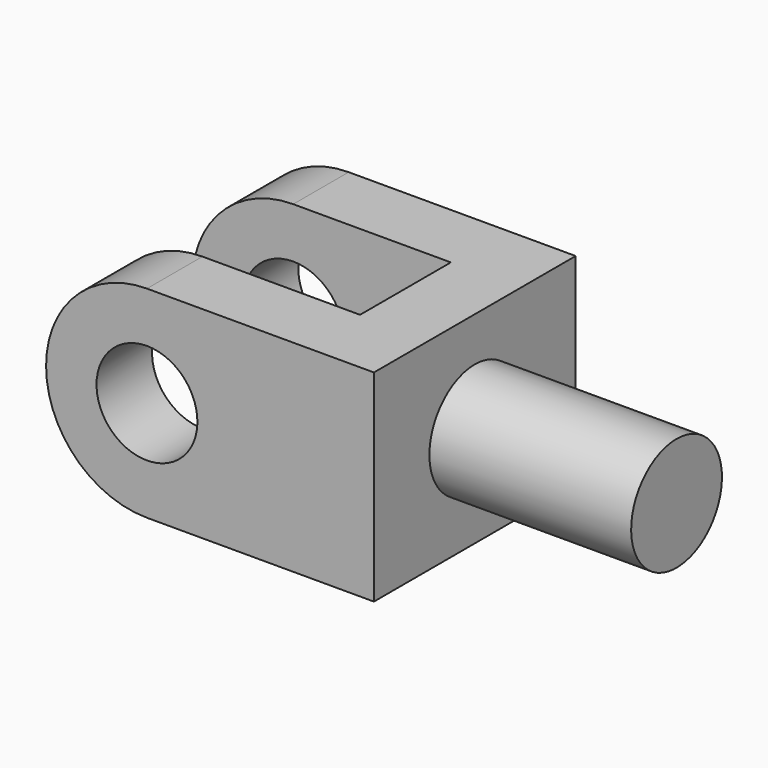
from build123d import *

# Parameters (mm, degrees)
F1_DEPTH = 812.8
F3_DEPTH = 1016.001
F4_R     = 406.4
F5_R     = 406.39999
F7_DEPTH = 812.8


# Not quite as in the source:
# - a fillet or chamfer is up to 0.001 mm smaller than in the source, because OpenCascade refuses the exact size


with BuildPart() as f1:
    # F0 (on Top) → F1 (new body)
    with BuildSketch(Plane.XY):
        Polygon((1205.200382638, 51.7077632248), (-115.599617362, 51.7077632248), (-115.599617362, -227.6922367752), (925.800382638, -227.6922367752), (925.800382638, -684.8922367752), (-115.599617362, -684.8922367752), (-115.599617362, -964.2922367752), (1205.200382638, -964.2922367752), (1205.200382638, -227.6922367752), align=None)
    extrude(amount=-F1_DEPTH)

    # F2 (on face) → F3 (cut, through all)
    with BuildSketch(Plane.XZ.offset(964.2922367752)):
        with BuildLine():
            ThreePointArc((494.000382638, -406.4), (434.4844805751, -262.7159020629), (290.800382638, -203.2))
            ThreePointArc((290.800382638, -203.2), (147.1162847009, -550.0840979371), (494.000382638, -406.4))
        make_face()
    extrude(amount=-F3_DEPTH, mode=Mode.SUBTRACT)

    # F4
    f4_edges = [f1.edges().sort_by_distance(p)[0] for p in [
        (-115.599617, -87.992237, 0),
        (-115.599617, -824.592237, 0),
    ]]
    fillet(f4_edges, radius=F4_R)

    # F5 (radius 406.4 in the source; OpenCascade refuses exactly that, so slightly less here)
    f5_edges = [f1.edges().sort_by_distance(p)[0] for p in [
        (-115.599617, -87.992237, -812.8),
        (-115.599617, -824.592237, -812.8),
    ]]
    fillet(f5_edges, radius=F5_R)

    # F6 (on face) → F7 (join)
    with BuildSketch(Plane.YZ.offset(1205.200382638)):
        with BuildLine():
            ThreePointArc((-227.6922367752, -406.4), (-294.6476265959, -244.7553898208), (-456.2922367752, -177.8))
            ThreePointArc((-456.2922367752, -177.8), (-617.9368469544, -568.0446101792), (-227.6922367752, -406.4))
        make_face()
    extrude(amount=F7_DEPTH)


solid = f1.part
